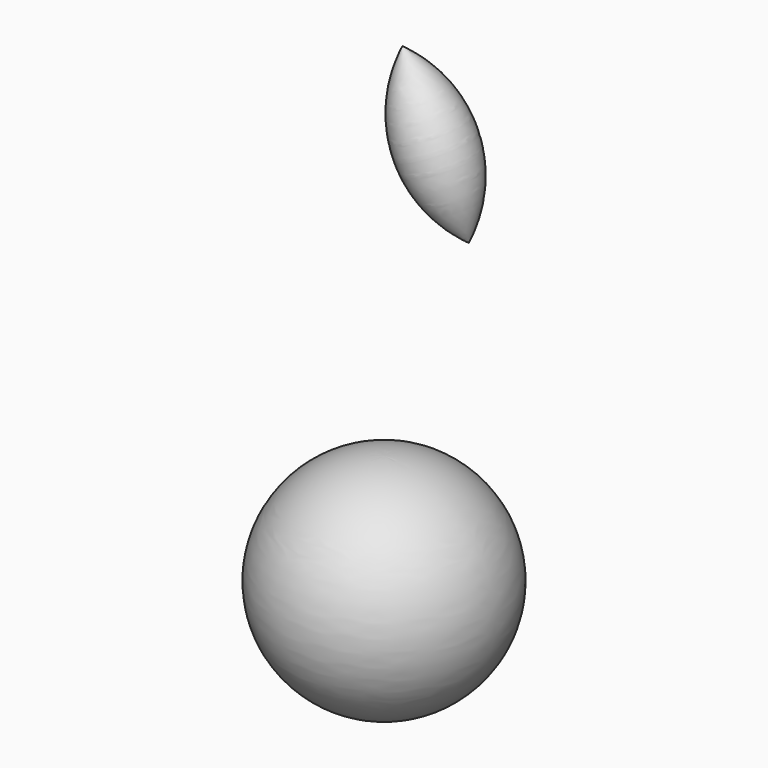
from build123d import *


with BuildPart() as f1:
    # F0 (on Front) → F1 (revolve)
    with BuildSketch(Plane.XZ):
        with BuildLine():
            Line((-21.3311258703, 24.5778430253), (-33.5632674396, 52.5370240211))
            ThreePointArc((-33.5632674396, 52.5370240211), (-33.3770086376, 35.9631408055), (-21.3311258703, 24.5778430253))
        make_face()
    revolve(axis=Axis((-27.447196655, 0, 38.5574335232), (0.4008188308, 0, -0.9161573363)))


with BuildPart() as f3:
    # F2 (on Front) → F3 (revolve)
    with BuildSketch(Plane.XZ):
        with BuildLine():
            Line((-36.9504876435, -15.0728514418), (-36.9504876435, -55.6002119509))
            ThreePointArc((-36.9504876435, -55.6002119509), (-16.577191664, -35.3365316963), (-36.9504876435, -15.0728514418))
        make_face()
    revolve(axis=Axis((-36.9504876435, 0, -35.0709706545), (0, 0, -1)))


solid = Compound([f1.part, f3.part])
